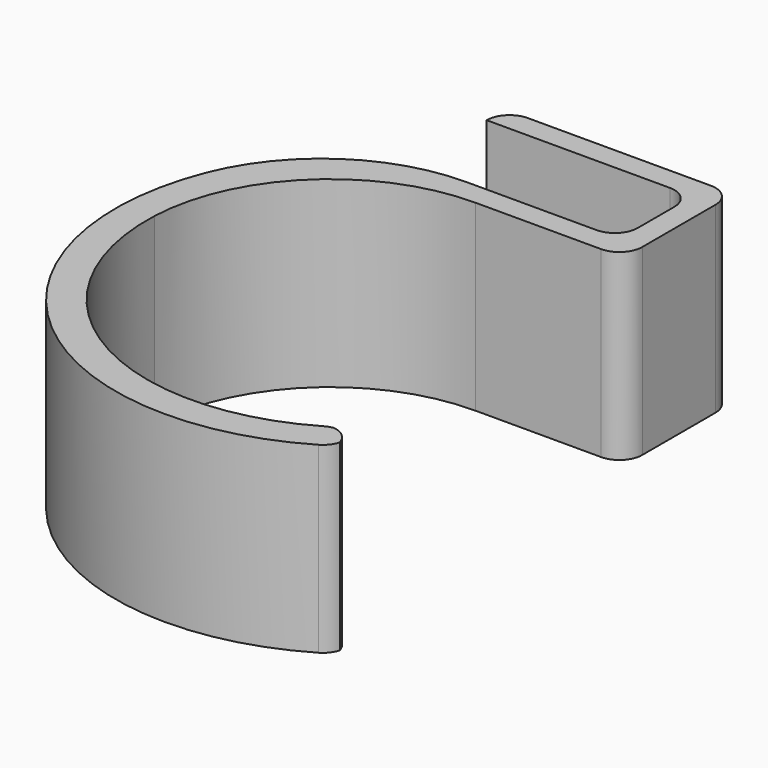
from build123d import *

# Parameters (mm, degrees)
F0_W        = 45
F0_H        = 5
F1_DEPTH    = 40
F2_T1_DEPTH = 40
F2_T3_DEPTH = 65
F2_T5_DEPTH = 54.4889687993
F2_T7_DEPTH = 46.9752871377
F3_R        = 39.6889865909


# Not quite as in the source:
# - a fillet or chamfer that OpenCascade refuses, or shapes differently, is made with other operations: its cross-section is extruded or revolved along the edge and cut away or added


with BuildPart() as f1:
    # F0 (on Top) → F1 (new body)
    with BuildSketch(Plane.XY):
        with Locations((27.5, 13.2681977808)):
            Rectangle(F0_W, F0_H)
        with BuildLine():
            Line((50, 10.7681977808), (50, -3.9824241135))
            ThreePointArc((50, -3.9824241135), (52.5291420669, -5.0643561015), (55, -6.273486986))
            Line((55, -6.273486986), (55, 15.7681977808))
            Line((55, 15.7681977808), (50, 15.7681977808))
            Line((50, 15.7681977808), (50, 10.7681977808))
        make_face()
        with BuildLine():
            ThreePointArc((55, -6.273486986), (52.5291420669, -5.0643561015), (50, -3.9824241135))
            Line((50, -3.9824241135), (50, -9.2318022192))
            Line((50, -9.2318022192), (50, -11.5117834926))
            ThreePointArc((50, -11.5117834926), (52.5410653135, -12.7963056669), (55, -14.2318022192))
            Line((55, -14.2318022192), (55, -6.273486986))
        make_face()
        with BuildLine():
            Line((15.8578643763, -9.2318022192), (5, -9.2318022192))
            Line((5, -9.2318022192), (5, -14.2318022192))
            ThreePointArc((5, -14.2318022192), (10.2699038194, -11.3864605272), (15.8578643763, -9.2318022192))
        make_face()
        with BuildLine():
            Line((5, -14.2318022192), (5, -9.2318022192))
            Line((5, -9.2318022192), (0, -9.2318022192))
            ThreePointArc((0, -9.2318022192), (-15, -84.2318022192), (60, -99.2318022192))
            Line((60, -99.2318022192), (60, -94.2318022192))
            Line((60, -94.2318022192), (55, -94.2318022192))
            ThreePointArc((55, -94.2318022192), (-10, -79.2318022192), (5, -14.2318022192))
        make_face()
        with BuildLine():
            ThreePointArc((15.8578643763, -9.2318022192), (10.2699038194, -11.3864605272), (5, -14.2318022192))
            Line((5, -14.2318022192), (50, -14.2318022192))
            Line((50, -14.2318022192), (50, -11.5117834926))
            ThreePointArc((50, -11.5117834926), (47.1090892478, -10.2741059066), (44.1421356237, -9.2318022192))
            Line((44.1421356237, -9.2318022192), (15.8578643763, -9.2318022192))
        make_face()
        with BuildLine():
            Line((50, -9.2318022192), (44.1421356237, -9.2318022192))
            ThreePointArc((44.1421356237, -9.2318022192), (47.1090892478, -10.2741059066), (50, -11.5117834926))
            Line((50, -11.5117834926), (50, -9.2318022192))
        make_face()
        with BuildLine():
            Line((50, -11.5117834926), (50, -14.2318022192))
            Line((50, -14.2318022192), (55, -14.2318022192))
            ThreePointArc((55, -14.2318022192), (52.5410653135, -12.7963056669), (50, -11.5117834926))
        make_face()
    extrude(amount=F1_DEPTH)

    # F2: fillet of radius 5 on 8 edges, made by hand

    # F2_s2 → F2_t1 (join)
    with BuildSketch(Plane.XY):
        with BuildLine():
            ThreePointArc((50, -4.2318022192), (48.5355339059, -7.7673361251), (45, -9.2318022192))
            Line((45, -9.2318022192), (50, -9.2318022192))
            Line((50, -9.2318022192), (50, -4.2318022192))
        make_face()
        with BuildLine():
            ThreePointArc((45, 10.7681977808), (48.5355339059, 9.3037316868), (50, 5.7681977808))
            Line((50, 5.7681977808), (50, 10.7681977808))
            Line((50, 10.7681977808), (45, 10.7681977808))
        make_face()
    extrude(amount=F2_T1_DEPTH)

    # F2_s4 → F2_t3 (cut)
    with BuildSketch(Plane.XY.offset(-12.5)):
        with BuildLine():
            ThreePointArc((55, -9.2318022192), (53.5355339059, -12.7673361251), (50, -14.2318022192))
            Line((50, -14.2318022192), (55, -14.2318022192))
            Line((55, -14.2318022192), (55, -9.2318022192))
        make_face()
        with BuildLine():
            ThreePointArc((50, 15.7681977808), (53.5355339059, 14.3037316868), (55, 10.7681977808))
            Line((55, 10.7681977808), (55, 15.7681977808))
            Line((55, 15.7681977808), (50, 15.7681977808))
        make_face()
        with BuildLine():
            ThreePointArc((5, 10.7681977808), (6.4644660941, 14.3037316868), (10, 15.7681977808))
            Line((10, 15.7681977808), (5, 15.7681977808))
            Line((5, 15.7681977808), (5, 10.7681977808))
        make_face()
        with BuildLine():
            ThreePointArc((60, -99.2318022192), (58.5355339059, -95.6962683132), (55, -94.2318022192))
            Line((55, -94.2318022192), (60, -94.2318022192))
            Line((60, -94.2318022192), (60, -99.2318022192))
        make_face()
    extrude(amount=F2_T3_DEPTH, mode=Mode.SUBTRACT)

    # F2_s6 → F2_t5 (cut)
    with BuildSketch(Plane.XY.offset(-7.2444843997)):
        with BuildLine():
            ThreePointArc((57.546692635, -100.7740381439), (59.3435851077, -98.9477505529), (60, -96.4712069105))
            Line((60, -96.4712069105), (60, -99.2318022192))
            ThreePointArc((60, -99.2318022192), (58.7836773401, -100.019354226), (57.546692635, -100.7740381439))
        make_face()
    extrude(amount=F2_T5_DEPTH, mode=Mode.SUBTRACT)

    # F2_s8 → F2_t7 (cut)
    with BuildSketch(Plane.XY.offset(-3.4876435688)):
        with BuildLine():
            ThreePointArc((56.3950574275, -94.2318022192), (55.0843622501, -94.4066516358), (53.8653367875, -94.9189709584))
            ThreePointArc((53.8653367875, -94.9189709584), (54.4350841017, -94.5793754416), (55, -94.2318022192))
            Line((55, -94.2318022192), (56.3950574275, -94.2318022192))
        make_face()
    extrude(amount=F2_T7_DEPTH, mode=Mode.SUBTRACT)

    # F3
    f3_edges = [f1.edges().sort_by_distance(p)[0] for p in [
        (0, -9.231802, 20),
        (5, -14.231802, 20),
    ]]
    fillet(f3_edges, radius=F3_R)


solid = f1.part
